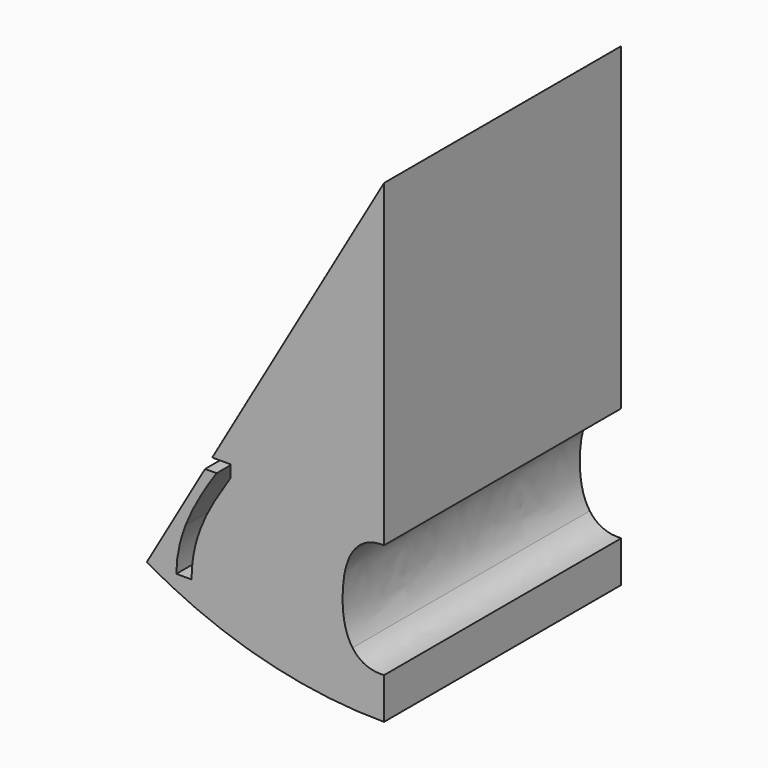
from build123d import *

# Parameters (mm, degrees)
F1_DEPTH = 25


# Not quite as in the source:
# - the program builds the solid bodies; features that only make, move or delete a surface that nothing else refers to are left out


with BuildPart() as f1:
    # F0 (on Front) → F1 (new body)
    with BuildSketch(Plane.XZ):
        with BuildLine():
            ThreePointArc((-20, -34.6410161514), (-10.3527618041, -38.6370330516), (0, -40))
            Line((0, -40), (0, -36.5303086516))
            add(Edge.make_bspline(
                [(0, -36.5303086516), (-0.1149220611, -36.5363907695), (-0.234185262, -36.5363907695)],
                knots=[0.9158257876, 0.9158257876, 0.9158257876, 1, 1, 1], degree=2))
            add(Edge.make_bspline(
                [(-0.234185262, -36.5363907695), (-1.8148580784, -36.5363907695), (-2.6530614293, -35.3588639809)],
                knots=[0, 0, 0, 1, 1, 1], degree=2))
            add(Edge.make_bspline(
                [(-2.6530614293, -35.3588639809), (-3.4912647801, -34.1813371924), (-3.4912647801, -31.9347820187)],
                knots=[0, 0, 0, 1, 1, 1], degree=2))
            add(Edge.make_bspline(
                [(-3.4912647801, -31.9347820187), (-3.4912647801, -29.5010139137), (-2.6200864243, -28.1979693646)],
                knots=[0, 0, 0, 1, 1, 1], degree=2))
            add(Edge.make_bspline(
                [(-2.6200864243, -28.1979693646), (-1.7489080686, -26.8949248154), (-0.1405787965, -26.8949248154)],
                knots=[0, 0, 0, 1, 1, 1], degree=2))
            add(Edge.make_bspline(
                [(-0.1405787965, -26.8949248154), (-0.0694054692, -26.8949248154), (0, -26.8970735535)],
                knots=[0, 0, 0, 0.0335559038, 0.0335559038, 0.0335559038], degree=2))
            Line((0, -26.8970735535), (0, 0))
            Line((0, 0), (-14.4835999879, -25.0863310555))
            Line((-14.4835999879, -25.0863310555), (-12.9261437307, -25.0863310555))
            Line((-12.9261437307, -25.0863310555), (-12.9261437307, -26.0823037829))
            add(Edge.make_bspline(
                [(-12.9261437307, -26.0823037829), (-14.4004454653, -28.334163173), (-15.0087314402, -29.6107992676)],
                knots=[0, 0, 0, 1, 1, 1], degree=2))
            add(Edge.make_bspline(
                [(-15.0087314402, -29.6107992676), (-15.6170174151, -30.8874353622), (-15.9206143649, -32.1302171206)],
                knots=[0, 0, 0, 1, 1, 1], degree=2))
            add(Edge.make_bspline(
                [(-15.9206143649, -32.1302171206), (-16.2242113147, -33.3729988791), (-16.2242113147, -34.7031466663)],
                knots=[0, 0, 0, 1, 1, 1], degree=2))
            Line((-16.2242113147, -34.7031466663), (-17.5063077861, -34.7031466663))
            add(Edge.make_bspline(
                [(-17.5063077861, -34.7031466663), (-17.5063077861, -32.8597234604), (-16.7254739044, -30.823002916)],
                knots=[0, 0, 0, 1, 1, 1], degree=2))
            add(Edge.make_bspline(
                [(-16.7254739044, -30.823002916), (-15.9446400228, -28.7862823716), (-14.1143217212, -26.1303550987)],
                knots=[0, 0, 0, 1, 1, 1], degree=2))
            Line((-14.1143217212, -26.1303550987), (-15.0863675502, -26.1303550987))
            Line((-15.0863675502, -26.1303550987), (-20, -34.6410161514))
        make_face()
    extrude(amount=F1_DEPTH)


solid = f1.part
